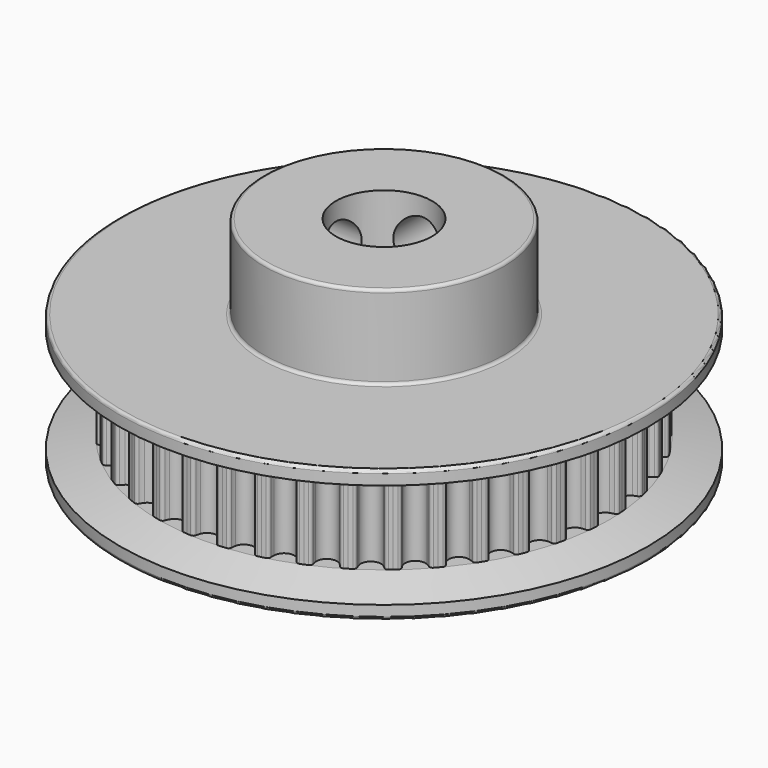
from build123d import *

# Parameters (mm, degrees)
F3_DEPTH    = 3.5
F4_COUNT    = 40
F5_R        = 22
F6_DEPTH    = 2
F7_R        = 22
F8_DEPTH    = 2
F9_R        = 10
F10_DEPTH   = 7
F11_R       = 4
F12_DEPTH   = 18.001
F13_R       = 2
F14_DEPTH   = 22.001
F15_R       = 2
F16_DEPTH   = 22.001
F17_SIZE2   = 0.8708348754
F17_SIZE    = 3.25
F17_2_SIZE2 = 0.8708348754
F17_2_SIZE  = 3.25
F18_R       = 0.25


# Not quite as in the source:
# - a feature names something its author has since deleted; it is built from what else it names


with BuildPart() as f3:
    # F2 (on Top) → F3 (new body, symmetric)
    with BuildSketch(Plane.XY):
        with BuildLine():
            ThreePointArc((0.7975372115, 18.1335958983), (0.4861081763, 17.7303135708), (0, 17.577593171))
            ThreePointArc((0, 17.577593171), (-0.4861081763, 17.7303135708), (-0.7975372115, 18.1335958983))
            ThreePointArc((-0.7975372115, 18.1335958983), (-0.8543507962, 18.2997412789), (-0.891624198, 18.471330219))
            ThreePointArc((-0.891624198, 18.471330219), (-0.98206772, 18.6274037538), (-1.1539973748, 18.6819855523))
            ThreePointArc((-1.1539973748, 18.6819855523), (-1.3113279306, 18.6716017838), (-1.4685654344, 18.659893078))
            Line((-1.4685654344, 18.659893078), (0, 0))
            Line((0, 0), (1.4685654344, 18.659893078))
            ThreePointArc((1.4685654344, 18.659893078), (1.3113279306, 18.6716017838), (1.1539973748, 18.6819855523))
            ThreePointArc((1.1539973748, 18.6819855523), (0.98206772, 18.6274037538), (0.891624198, 18.471330219))
            ThreePointArc((0.891624198, 18.471330219), (0.8543507962, 18.2997412789), (0.7975372115, 18.1335958983))
        make_face()
    extrude(amount=F3_DEPTH, both=True)

    # F4: F3 ×40 about axis
    f4_axis = Axis((0, 0, 0), (0, 0, -1))


with BuildPart() as f3_1:
    add(f3.part)
    for i in range(1, F4_COUNT):
        add(f3.part.rotate(f4_axis, i * 360 / F4_COUNT))

    # F5 (on face) → F6 (join)
    with BuildSketch(Plane(origin=(0, 0, -3.5), x_dir=(1, 0, 0), z_dir=(0, 0, -1))):
        Circle(F5_R)
    extrude(amount=F6_DEPTH)

    # F7 (on face) → F8 (join)
    with BuildSketch(Plane.XY.offset(3.5)):
        Circle(F7_R)
    extrude(amount=F8_DEPTH)

    # F9 (on face) → F10 (join)
    with BuildSketch(Plane.XY.offset(5.5)):
        Circle(F9_R)
    extrude(amount=F10_DEPTH)

    # F11 (on face) → F12 (cut, through all)
    with BuildSketch(Plane.XY.offset(12.5)):
        Circle(F11_R)
    extrude(amount=-F12_DEPTH, mode=Mode.SUBTRACT)

    # F13 (on Front) → F14 (cut, through all)
    with BuildSketch(Plane.XZ):
        with Locations((0, 9)):
            Circle(F13_R)
    extrude(amount=-F14_DEPTH, mode=Mode.SUBTRACT)

    # F15 (on Right) → F16 (cut, through all)
    with BuildSketch(Plane.YZ):
        with Locations((0, 9)):
            Circle(F15_R)
    extrude(amount=-F16_DEPTH, mode=Mode.SUBTRACT)

    # F17
    f17_edges = [f3_1.edges().sort_by_distance(p)[0] for p in [
        (-22, 0, -3.5),
    ]]
    f17_side = f3_1.faces().sort_by_distance((-21.377746, 0, -3.5))[0]
    chamfer(f17_edges, length=F17_SIZE, length2=F17_SIZE2, reference=f17_side)

    # F17#2
    f17_2_edges = [f3_1.edges().sort_by_distance(p)[0] for p in [
        (-22, 0, 3.5),
    ]]
    f17_2_side = f3_1.faces().sort_by_distance((-21.377746, 0, 3.5))[0]
    chamfer(f17_2_edges, length=F17_2_SIZE, length2=F17_2_SIZE2, reference=f17_2_side)

    # F18
    f18_edges = [f3_1.edges().sort_by_distance(p)[0] for p in [
        (-10, 0, 5.5),
        (-10, 0, 12.5),
        (-22, 0, 5.5),
        (-22, 0, -5.5),
    ]]
    fillet(f18_edges, radius=F18_R)


solid = f3_1.part
